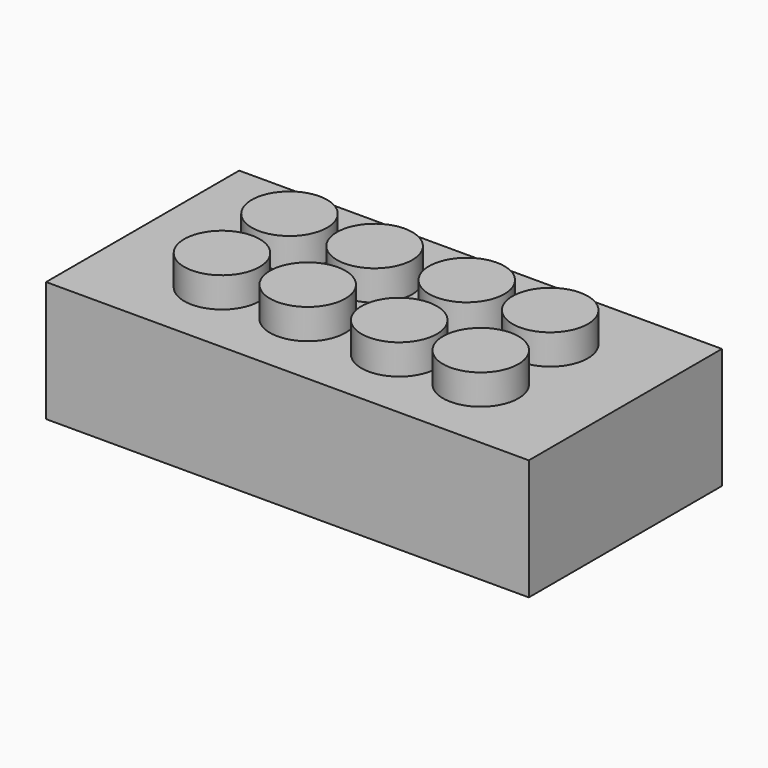
from build123d import *

# Parameters (mm, degrees)
F0_W     = 32
F0_H     = 16
F1_DEPTH = 8
F3_R     = 2.5
F4_DEPTH = 2
F5_T     = -1


# Not quite as in the source:
# - the program builds the solid bodies; features that only make, move or delete a surface that nothing else refers to are left out


with BuildPart() as f1:
    # F0 (on Top) → F1 (new body)
    with BuildSketch(Plane.XY):
        with Locations((0.0749295065, 8)):
            Rectangle(F0_W, F0_H)
    extrude(amount=F1_DEPTH)

    # F3 (on offset) → F4 (join)
    with BuildSketch(Plane.XY.offset(8)):
        with Locations((-8.4686602995, 10.8479883277)):
            Circle(F3_R)
        with Locations((-2.7646990493, 10.774385184)):
            Circle(F3_R)
        with Locations((3.3415844664, 10.774385184)):
            Circle(F3_R)
        with Locations((8.8161835447, 10.8445733786)):
            Circle(F3_R)
        with Locations((8.8161835447, 5.0892247818)):
            Circle(F3_R)
        with Locations((3.4117714968, 5.0892247818)):
            Circle(F3_R)
        with Locations((-2.7646990493, 5.2295993082)):
            Circle(F3_R)
        with Locations((-8.4498599172, 5.2295993082)):
            Circle(F3_R)
    extrude(amount=F4_DEPTH)

    # F5
    f5_openings = [f1.faces().sort_by_distance(p)[0] for p in [
        (0.07493, 8, 0),
    ]]
    offset(amount=F5_T, openings=f5_openings, kind=Kind.INTERSECTION)


solid = f1.part
